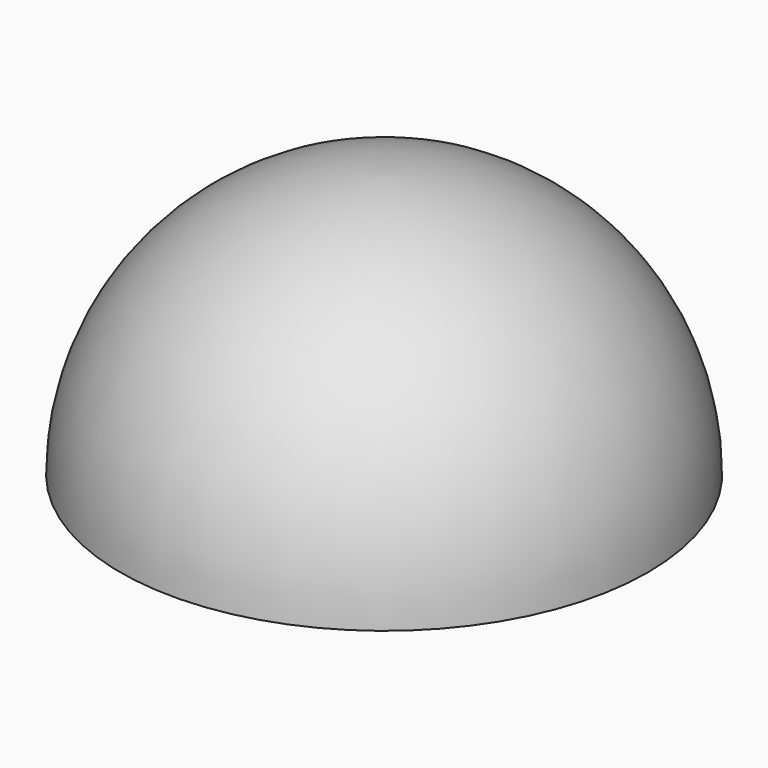
from build123d import *

# Parameters (mm, degrees)
F0_R     = 25.4
F1_DEPTH = 25.4
F2_R     = 25.39999


# Not quite as in the source:
# - a fillet or chamfer is up to 0.001 mm smaller than in the source, because OpenCascade refuses the exact size


with BuildPart() as f1:
    # F0 (on Top) → F1 (new body)
    with BuildSketch(Plane.XY):
        Circle(F0_R)
    extrude(amount=F1_DEPTH)

    # F2 (radius 25.4 in the source; OpenCascade refuses exactly that, so slightly less here)
    f2_edges = [f1.edges().sort_by_distance(p)[0] for p in [
        (-25.4, 0, 25.4),
    ]]
    fillet(f2_edges, radius=F2_R)


solid = f1.part
